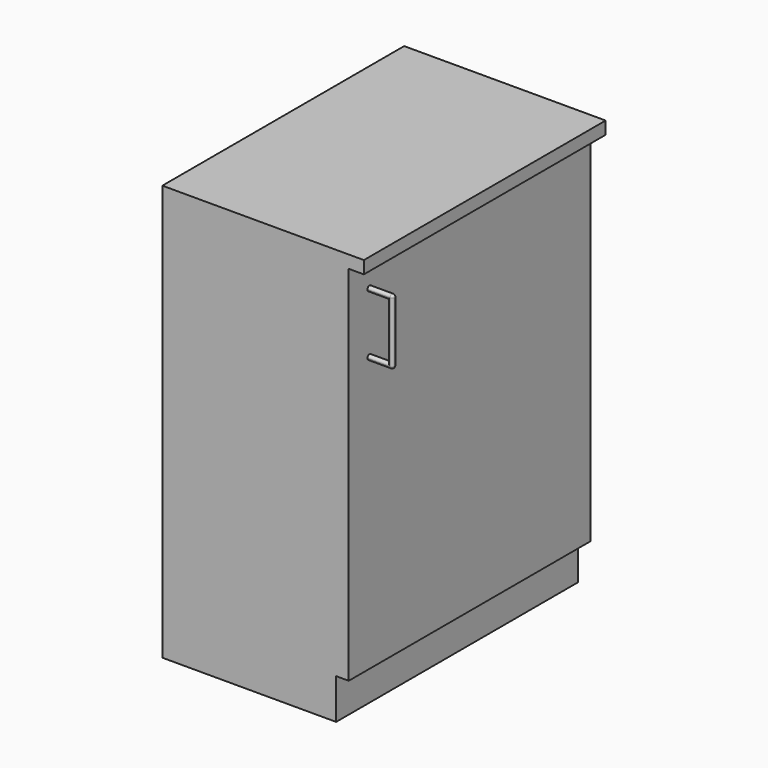
from build123d import *

# Parameters (mm, degrees)
F0_W        = 370
F0_H        = 600
F1_DEPTH    = 800
F2_W        = 600
F2_H        = 80
F3_DEPTH    = 25
F5_DEPTH    = 50
F6_T1_DEPTH = 120
F6_T4_ANGLE = 180
F6_T6_ANGLE = 180
F7_W        = 40
F7_H        = 110
F8_DEPTH    = 25
F9_R        = 4.99999
F10_W       = 400
F10_H       = 600
F11_DEPTH   = 25


# Not quite as in the source:
# - a fillet or chamfer that OpenCascade refuses, or shapes differently, is made with other operations: its cross-section is extruded or revolved along the edge and cut away or added
# - a fillet or chamfer is up to 0.001 mm smaller than in the source, because OpenCascade refuses the exact size


with BuildPart() as f1:
    # F0 (on Top) → F1 (new body)
    with BuildSketch(Plane.XY):
        Rectangle(F0_W, F0_H)
    extrude(amount=F1_DEPTH)

    # F2 (on face) → F3 (cut)
    with BuildSketch(Plane.YZ.offset(185)):
        with Locations((0, 40)):
            Rectangle(F2_W, F2_H)
    extrude(amount=-F3_DEPTH, mode=Mode.SUBTRACT)

    # F4 (on face) → F5 (join)
    with BuildSketch(Plane.YZ.offset(185)):
        with BuildLine():
            ThreePointArc((-248.5795542598, 750), (-252.1150881657, 748.5355339059), (-253.5795542598, 745))
            Line((-253.5795542598, 745), (-253.5795542598, 625))
            ThreePointArc((-253.5795542598, 625), (-252.1150881657, 621.4644660941), (-248.5795542598, 620))
            ThreePointArc((-248.5795542598, 620), (-245.0440203538, 621.4644660941), (-243.5795542598, 625))
            Line((-243.5795542598, 625), (-243.5795542598, 745))
            ThreePointArc((-243.5795542598, 745), (-245.0440203538, 748.5355339059), (-248.5795542598, 750))
        make_face()
    extrude(amount=F5_DEPTH)

    # F6: fillet of radius 5 on 4 edges, made by hand

    # F6_s2 → F6_t1 (cut)
    with BuildSketch(Plane.XY.offset(625)):
        with BuildLine():
            ThreePointArc((230, -253.5795542598), (233.5355339059, -252.1150881657), (235, -248.5795542598))
            Line((235, -248.5795542598), (235, -253.5795542598))
            Line((235, -253.5795542598), (230, -253.5795542598))
        make_face()
        with BuildLine():
            ThreePointArc((230, -243.5795542598), (233.5355339059, -245.0440203538), (235, -248.5795542598))
            Line((235, -248.5795542598), (235, -243.5795542598))
            Line((235, -243.5795542598), (230, -243.5795542598))
        make_face()
    extrude(amount=F6_T1_DEPTH, mode=Mode.SUBTRACT)

    # F6_s3 → F6_t4 (revolve, cut)
    with BuildSketch(Plane.XY.offset(745)):
        with BuildLine():
            ThreePointArc((230, -253.5795542598), (233.5355339059, -252.1150881657), (235, -248.5795542598))
            Line((235, -248.5795542598), (235, -253.5795542598))
            Line((235, -253.5795542598), (230, -253.5795542598))
        make_face()
    revolve(axis=Axis((235, -248.5795542598, 745), (-1, 0, 0)), revolution_arc=F6_T4_ANGLE, mode=Mode.SUBTRACT)

    # F6_s5 → F6_t6 (revolve, cut)
    with BuildSketch(Plane.XY.offset(625)):
        with BuildLine():
            ThreePointArc((230, -243.5795542598), (233.5355339059, -245.0440203538), (235, -248.5795542598))
            Line((235, -248.5795542598), (235, -243.5795542598))
            Line((235, -243.5795542598), (230, -243.5795542598))
        make_face()
    revolve(axis=Axis((235, -248.5795542598, 625), (-1, 0, 0)), revolution_arc=F6_T6_ANGLE, mode=Mode.SUBTRACT)

    # F7 (on face) → F8 (cut)
    with BuildSketch(Plane(origin=(0, -243.5795542598, 0), x_dir=(-1, 0, 0), z_dir=(0, 1, 0))):
        with Locations((-205, 685)):
            Rectangle(F7_W, F7_H)
    extrude(amount=-F8_DEPTH, mode=Mode.SUBTRACT)

    # F9 (radius 5 in the source; OpenCascade refuses exactly that, so slightly less here)
    f9_edges = [f1.edges().sort_by_distance(p)[0] for p in [
        (205, -243.579554, 740),
        (225, -243.579554, 685),
        (205, -243.579554, 630),
        (205, -253.579554, 740),
        (225, -253.579554, 685),
        (205, -253.579554, 630),
    ]]
    fillet(f9_edges, radius=F9_R)

    # F10 (on face) → F11 (join)
    with BuildSketch(Plane.XY.offset(800)):
        with Locations((15, 0)):
            Rectangle(F10_W, F10_H)
    extrude(amount=F11_DEPTH)


solid = f1.part
